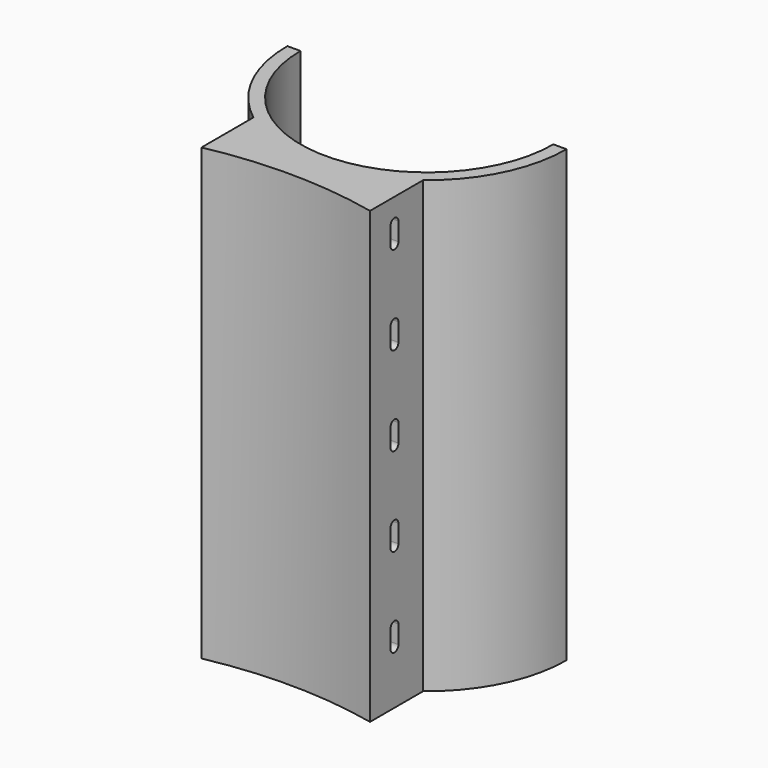
from build123d import *
from build123d import SkipClean  # not in build123d's __all__

# Parameters (mm, degrees)
F0_R      = 42.5
F1_DEPTH  = 7
F2_R      = 15
F3_DEPTH  = 25
F4_R      = 42.5
F4_R_2    = 38.5
F5_DEPTH  = 130
F7_DEPTH  = 130
F9_DEPTH  = 137.001
F11_DEPTH = 137
F13_DEPTH = 68.3435688744


with BuildPart() as f1:
    # F0 (on Top) → F1 (new body)
    with BuildSketch(Plane.XY):
        Circle(F0_R)
    extrude(amount=F1_DEPTH)

    # F2 (on face) → F3 (cut)
    with BuildSketch(Plane.XY.offset(7)):
        Circle(F2_R)
    extrude(amount=-F3_DEPTH, mode=Mode.SUBTRACT)

    # F4 (on face) → F5 (join)
    with BuildSketch(Plane.XY.offset(7)):
        Circle(F4_R)
        Circle(F4_R_2, mode=Mode.SUBTRACT)
    extrude(amount=F5_DEPTH)

    # F6 (on face) → F7 (cut, through all)
    with BuildSketch(Plane.XY.offset(137)):
        with BuildLine():
            ThreePointArc((-36.1781659003, 13.167775518), (-27.2236110757, 27.2236110757), (-13.167775518, 36.1781659003))
            Line((-13.167775518, 36.1781659003), (-14.5358560913, 39.9369363834))
            ThreePointArc((-14.5358560913, 39.9369363834), (-30.0520382004, 30.0520382004), (-39.9369363834, 14.5358560913))
            Line((-39.9369363834, 14.5358560913), (-36.1781659003, 13.167775518))
        make_face()
        with BuildLine():
            Line((0, 0), (0, 38.5))
            ThreePointArc((0, 38.5), (-6.6854548402, 37.915098491), (-13.167775518, 36.1781659003))
            ThreePointArc((-13.167775518, 36.1781659003), (-27.2236110757, 27.2236110757), (-36.1781659003, 13.167775518))
            ThreePointArc((-36.1781659003, 13.167775518), (-37.915098491, 6.6854548402), (-38.5, 0))
            Line((-38.5, 0), (0, 0))
        make_face()
        with BuildLine():
            ThreePointArc((0, 38.5), (6.6854548402, 37.915098491), (13.167775518, 36.1781659003))
            Line((13.167775518, 36.1781659003), (14.5358560913, 39.9369363834))
            ThreePointArc((14.5358560913, 39.9369363834), (7.3800475508, 41.854329503), (0, 42.5))
            Line((0, 42.5), (0, 38.5))
        make_face()
        with BuildLine():
            ThreePointArc((13.167775518, 36.1781659003), (27.2236110757, 27.2236110757), (36.1781659003, 13.167775518))
            Line((36.1781659003, 13.167775518), (39.9369363834, 14.5358560913))
            ThreePointArc((39.9369363834, 14.5358560913), (30.0520382004, 30.0520382004), (14.5358560913, 39.9369363834))
            Line((14.5358560913, 39.9369363834), (13.167775518, 36.1781659003))
        make_face()
    with SkipClean():  # cleaning this boolean's faces spoils the solid; the shape is the same uncleaned
        extrude(amount=-F7_DEPTH, mode=Mode.SUBTRACT)

    # F8 (on face) → F9 (cut, through all)
    with BuildSketch(Plane.XY.offset(137)):
        with BuildLine():
            ThreePointArc((-36.1781659003, 13.167775518), (-37.915098491, 6.6854548402), (-38.5, 0))
            Line((-38.5, 0), (38.5, 0))
            ThreePointArc((38.5, 0), (37.915098491, 6.6854548402), (36.1781659003, 13.167775518))
            Line((36.1781659003, 13.167775518), (39.9369363834, 14.5358560913))
            ThreePointArc((39.9369363834, 14.5358560913), (41.854329503, 7.3800475508), (42.5, 0))
            Line((42.5, 0), (48.543676734, 0))
            Line((48.543676734, 0), (48.543676734, 50.1251481473))
            Line((48.543676734, 50.1251481473), (-44.8859259486, 50.1251481473))
            Line((-44.8859259486, 50.1251481473), (-44.8859259486, 0))
            Line((-44.8859259486, 0), (-42.5, 0))
            ThreePointArc((-42.5, 0), (-41.854329503, 7.3800475508), (-39.9369363834, 14.5358560913))
            Line((-39.9369363834, 14.5358560913), (-36.1781659003, 13.167775518))
        make_face()
        with BuildLine():
            Line((-42.5, 0), (-38.5, 0))
            ThreePointArc((-38.5, 0), (-37.915098491, 6.6854548402), (-36.1781659003, 13.167775518))
            Line((-36.1781659003, 13.167775518), (-39.9369363834, 14.5358560913))
            ThreePointArc((-39.9369363834, 14.5358560913), (-41.854329503, 7.3800475508), (-42.5, 0))
        make_face()
        with BuildLine():
            ThreePointArc((36.1781659003, 13.167775518), (37.915098491, 6.6854548402), (38.5, 0))
            Line((38.5, 0), (42.5, 0))
            ThreePointArc((42.5, 0), (41.854329503, 7.3800475508), (39.9369363834, 14.5358560913))
            Line((39.9369363834, 14.5358560913), (36.1781659003, 13.167775518))
        make_face()
    extrude(amount=-F9_DEPTH, mode=Mode.SUBTRACT)

    # F10 (on face) → F11 (join, through all)
    with BuildSketch(Plane.XY.offset(137)):
        with BuildLine():
            ThreePointArc((25.8425688744, -33.7403561625), (0, -42.5), (-25.8425688744, -33.7403561625))
            Line((-25.8425688744, -33.7403561625), (-25.8425688744, -53.5076856613))
            ThreePointArc((-25.8425688744, -53.5076856613), (0.0246650595, -51.0317648548), (25.8425688744, -53.9779179117))
            Line((25.8425688744, -53.9779179117), (25.8425688744, -33.7403561625))
        make_face()
    extrude(amount=-F11_DEPTH)

    # F12 (on face) → F13 (cut, through all)
    with BuildSketch(Plane(origin=(-25.8425688744, 0, 0), x_dir=(0, -1, 0), z_dir=(-1, 0, 0))):
        with BuildLine():
            Line((46.1543562332, 124.3293995603), (46.1543562332, 129.8293995603))
            ThreePointArc((46.1543562332, 129.8293995603), (44.6543562332, 131.3293995603), (43.1543562332, 129.8293995603))
            Line((43.1543562332, 129.8293995603), (43.1543562332, 124.3293995603))
            ThreePointArc((43.1543562332, 124.3293995603), (44.6543562332, 122.8293995603), (46.1543562332, 124.3293995603))
        make_face()
        with BuildLine():
            Line((46.1543562332, 97.3293995603), (46.1543562332, 102.8293995603))
            ThreePointArc((46.1543562332, 102.8293995603), (44.6543562332, 104.3293995603), (43.1543562332, 102.8293995603))
            Line((43.1543562332, 102.8293995603), (43.1543562332, 97.3293995603))
            ThreePointArc((43.1543562332, 97.3293995603), (44.6543562332, 95.8293995603), (46.1543562332, 97.3293995603))
        make_face()
        with BuildLine():
            Line((46.1543562332, 70.3293995603), (46.1543562332, 75.8293995603))
            ThreePointArc((46.1543562332, 75.8293995603), (44.6543562332, 77.3293995603), (43.1543562332, 75.8293995603))
            Line((43.1543562332, 75.8293995603), (43.1543562332, 70.3293995603))
            ThreePointArc((43.1543562332, 70.3293995603), (44.6543562332, 68.8293995603), (46.1543562332, 70.3293995603))
        make_face()
        with BuildLine():
            Line((46.1543562332, 43.3293995603), (46.1543562332, 48.8293995603))
            ThreePointArc((46.1543562332, 48.8293995603), (44.6543562332, 50.3293995603), (43.1543562332, 48.8293995603))
            Line((43.1543562332, 48.8293995603), (43.1543562332, 43.3293995603))
            ThreePointArc((43.1543562332, 43.3293995603), (44.6543562332, 41.8293995603), (46.1543562332, 43.3293995603))
        make_face()
        with BuildLine():
            Line((46.1543562332, 16.3293995603), (46.1543562332, 21.8293995603))
            ThreePointArc((46.1543562332, 21.8293995603), (44.6543562332, 23.3293995603), (43.1543562332, 21.8293995603))
            Line((43.1543562332, 21.8293995603), (43.1543562332, 16.3293995603))
            ThreePointArc((43.1543562332, 16.3293995603), (44.6543562332, 14.8293995603), (46.1543562332, 16.3293995603))
        make_face()
    extrude(amount=-F13_DEPTH, mode=Mode.SUBTRACT)


solid = f1.part
